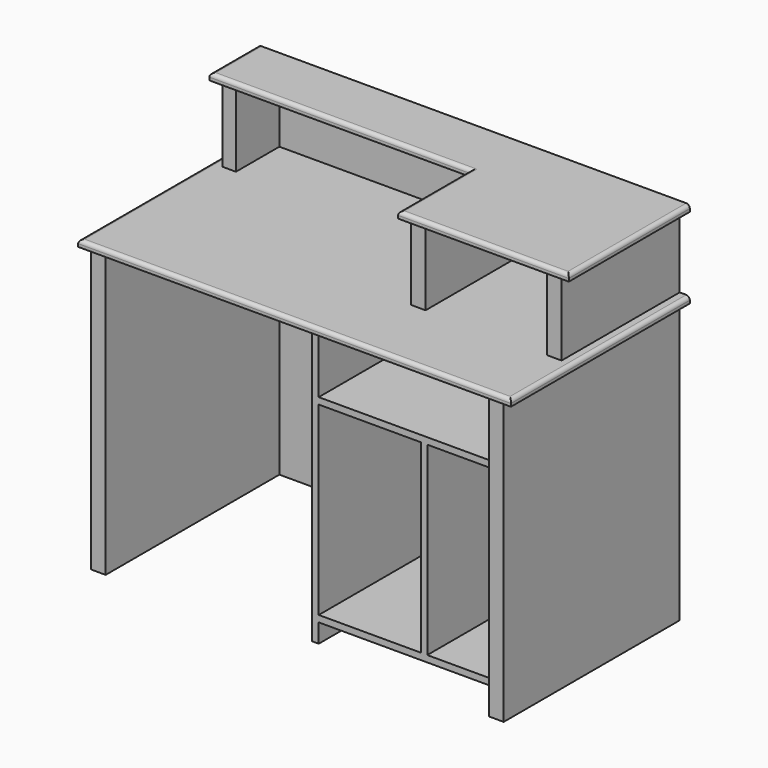
from build123d import *

# Parameters (mm, degrees)
F0_W      = 18
F0_H      = 564
F1_DEPTH  = 780
F2_W      = 18
F2_H      = 512
F3_DEPTH  = 564
F5_DEPTH  = 18
F6_R      = 10
F7_W      = 40
F7_H      = 250
F7_H_2    = 150
F8_DEPTH  = 205
F10_DEPTH = 18
F11_R     = 10


with BuildPart() as f1:
    # F0 (on Top) → F1 (new body)
    with BuildSketch(Plane.XY):
        Polygon((-40, 0), (0, 0), (0, 608), (-1140, 608), (-1140, 0), (-1100, 0), (-1100, 600), (-558, 600), (-540, 600), (-40, 600), align=None)
        with Locations((-549, 318)):
            Rectangle(F0_W, F0_H)
    extrude(amount=F1_DEPTH)

    # F2 (on face) → F3 (join)
    with BuildSketch(Plane.XZ.offset(-600)):
        Polygon((-540, 70), (-540, 52), (-40, 52), (-40, 70), (-240, 70), (-258, 70), align=None)
        with Locations((-249, 326)):
            Rectangle(F2_W, F2_H)
        Polygon((-540, 600), (-540, 582), (-258, 582), (-240, 582), (-40, 582), (-40, 600), align=None)
    extrude(amount=F3_DEPTH)

    # F4 (on face) → F5 (join)
    with BuildSketch(Plane.XY.offset(780)):
        Polygon((28, 608), (0, 608), (0, 0), (-40, 0), (-40, 600), (-540, 600), (-540, 36), (-558, 36), (-558, 600), (-1100, 600), (-1100, 0), (-1140, 0), (-1140, 608), (-1168, 608), (-1168, -10), (28, -10), align=None)
        Polygon((0, 0), (0, 608), (-1140, 608), (-1140, 0), (-1100, 0), (-1100, 600), (-558, 600), (-558, 36), (-540, 36), (-540, 600), (-40, 600), (-40, 0), align=None)
    extrude(amount=F5_DEPTH)

    # F6
    f6_edges = [f1.edges().sort_by_distance(p)[0] for p in [
        (-570, -10, 798),
        (-1168, 299, 798),
        (28, 299, 798),
    ]]
    fillet(f6_edges, radius=F6_R)

    # F7 (on face) → F8 (join)
    with BuildSketch(Plane.XY.offset(798)):
        Polygon((0, 450), (0, 608), (-40, 608), (-40, 600), (-40, 450), align=None)
        Polygon((-40, 600), (-40, 608), (-1100, 608), (-1100, 600), (-415.8988296986, 600), (-375.8988296986, 600), align=None)
        with Locations((-20, 325)):
            Rectangle(F7_W, F7_H)
        Polygon((-1100, 600), (-1100, 608), (-1137.470126152, 608), (-1137.470126152, 450), (-1100, 450), align=None)
        with Locations((-395.8988296986, 525)):
            Rectangle(F7_W, F7_H_2)
        with Locations((-395.8988296986, 325)):
            Rectangle(F7_W, F7_H)
    extrude(amount=F8_DEPTH)

    # F9 (on face) → F10 (join)
    with BuildSketch(Plane.XY.offset(1003)):
        Polygon((0, 608), (-1137.470126152, 608), (-1137.470126152, 450), (-1100, 450), (-1100, 600), (-415.8988296986, 600), (-415.8988296986, 200), (-375.8988296986, 200), (-375.8988296986, 600), (-40, 600), (-40, 200), (0, 200), align=None)
        Polygon((-1137.470126152, 450), (-1137.470126152, 608), (-1165.470126152, 608), (-1165.470126152, 440), (-443.8988296986, 440), (-443.8988296986, 190), (28, 190), (28, 608), (0, 608), (0, 200), (-40, 200), (-40, 600), (-375.8988296986, 600), (-375.8988296986, 200), (-415.8988296986, 200), (-415.8988296986, 600), (-1100, 600), (-1100, 450), align=None)
    extrude(amount=F10_DEPTH)

    # F11
    f11_edges = [f1.edges().sort_by_distance(p)[0] for p in [
        (-1165.470126, 524, 1021),
        (-804.684478, 440, 1021),
        (-443.89883, 315, 1021),
        (-207.949415, 190, 1021),
        (28, 399, 1021),
    ]]
    fillet(f11_edges, radius=F11_R)


solid = f1.part
